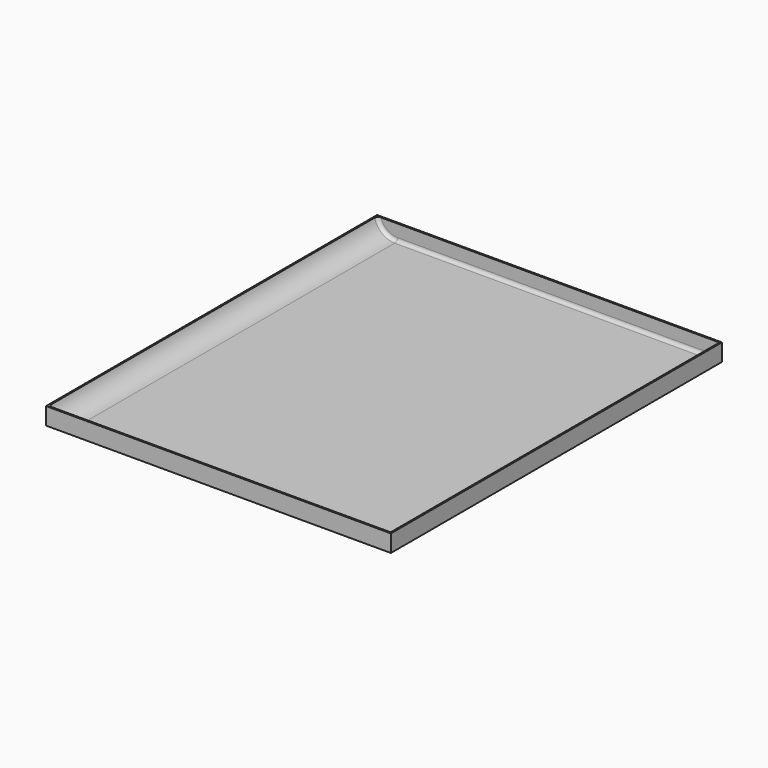
from build123d import *

# Parameters (mm, degrees)
F0_W        = 200
F0_H        = 240
F1_DEPTH    = 10
F2_T        = -0.8
F3_T1_DEPTH = 238.4
F4_R        = 2


# Not quite as in the source:
# - a fillet or chamfer that OpenCascade refuses, or shapes differently, is made with other operations: its cross-section is extruded or revolved along the edge and cut away or added


with BuildPart() as f1:
    # F0 (on Top) → F1 (new body)
    with BuildSketch(Plane.XY):
        with Locations((9.3512600348, 8.6151771247)):
            Rectangle(F0_W, F0_H)
    extrude(amount=F1_DEPTH)

    # F2
    f2_openings = [f1.faces().sort_by_distance(p)[0] for p in [
        (9.35126, 8.615177, 10),
    ]]
    offset(amount=F2_T, openings=f2_openings)

    # F3: fillet of radius 12 on 1 edges, made by hand

    # F3_s2 → F3_t1 (join)
    with BuildSketch(Plane.XZ.offset(-127.8151771247)):
        with BuildLine():
            ThreePointArc((-89.8487399652, 10), (-85.609648497, 3.3766248085), (-78.1799782486, 0.8))
            Line((-78.1799782486, 0.8), (-89.8487399652, 0.8))
            Line((-89.8487399652, 0.8), (-89.8487399652, 10))
        make_face()
    extrude(amount=F3_T1_DEPTH)

    # F4
    f4_edges = [f1.edges().sort_by_distance(p)[0] for p in [
        (15.185641, 127.815177, 0.8),
        (15.185641, -110.584823, 0.8),
        (108.55126, 8.615177, 0.8),
        (-85.609648, 127.815177, 3.376625),
        (-85.609648, -110.584823, 3.376625),
    ]]
    fillet(f4_edges, radius=F4_R)


solid = f1.part
